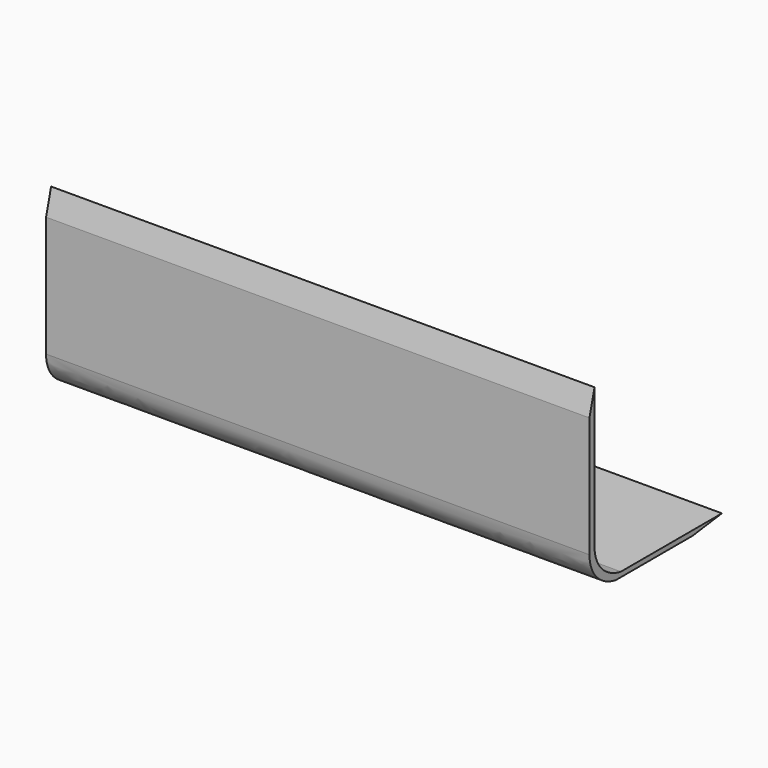
from build123d import *

# Parameters (mm, degrees)
F1_DEPTH = 254
F2_R     = 7.5365841045
F3_DEPTH = 25.4


# Not quite as in the source:
# - the program builds the solid bodies; features that only make, move or delete a surface that nothing else refers to are left out


with BuildPart() as f1:
    # F0 (on Right) → F1 (new body)
    with BuildSketch(Plane.YZ):
        with BuildLine():
            Line((2.9371477504, 67.7488154993), (0, 56.3350282609))
            Line((0, 56.3350282609), (0, 0))
            add(Edge.make_bspline(
                [(0, 0), (0, -8.9850798249), (6.8457759917, -15.2603751048), (15.4029959813, -16.6865773499)],
                knots=[0, 0, 0, 0, 22.7089002123, 22.7089002123, 22.7089002123, 22.7089002123], degree=3))
            Line((15.4029959813, -16.6865773499), (60.1857788861, -16.6865773499))
            Line((60.1857788861, -16.6865773499), (77.3849593316, -14.4004908129))
            Line((77.3849593316, -14.4004908129), (18.3401437317, -14.4004908129))
            add(Edge.make_bspline(
                [(2.9371477504, 2.286086537), (2.9371477504, -6.6989932879), (9.7829237421, -12.9742885678), (18.3401437317, -14.4004908129)],
                knots=[0, 0, 0, 0, 22.7089002123, 22.7089002123, 22.7089002123, 22.7089002123], degree=3))
            Line((2.9371477504, 2.286086537), (2.9371477504, 67.7488154993))
        make_face()
    extrude(amount=F1_DEPTH)

    # F2 (on face) → F3 (join)
    with BuildSketch(Plane(origin=(0, 2.9371477504, 0), x_dir=(-1, 0, 0), z_dir=(0, 1, 0))):
        with Locations((-11.9260810316, 33.5152037442)):
            Circle(F2_R)
    extrude(amount=F3_DEPTH)


solid = f1.part
